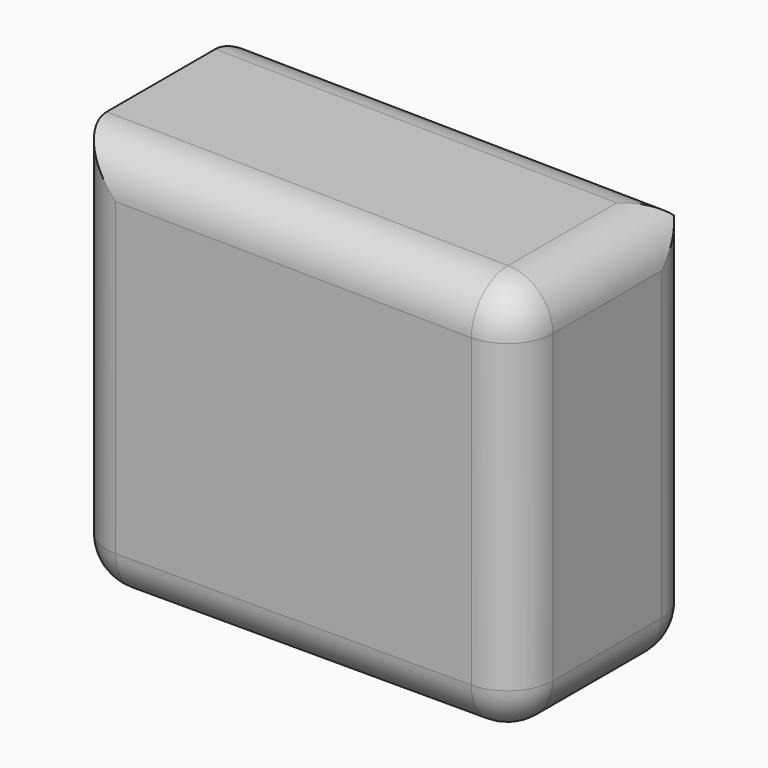
from build123d import *

# Parameters (mm, degrees)
F1_DEPTH    = 25.4
F2_R        = 5.08
F3_T1_DEPTH = 27.7897108637
F3_T6_DEPTH = 5.1816


# Not quite as in the source:
# - a fillet or chamfer that OpenCascade refuses, or shapes differently, is made with other operations: its cross-section is extruded or revolved along the edge and cut away or added


with BuildPart() as f1:
    # F0 (on Front) → F1 (new body)
    with BuildSketch(Plane.XZ):
        Polygon((-8.6416769773, 61.5346953273), (-58.7037988007, 62.1306672692), (-58.7037988007, 17.1343572438), (-8.6416769773, 17.1343572438), align=None)
    extrude(amount=F1_DEPTH)

    # F2
    f2_edges = [f1.edges().sort_by_distance(p)[0] for p in [
        (-33.672738, -25.4, 61.832681),
        (-58.703799, -25.4, 39.632512),
        (-33.672738, -25.4, 17.134357),
        (-8.641677, -25.4, 39.334526),
        (-33.672738, 0, 61.832681),
        (-58.703799, 0, 39.632512),
        (-33.672738, 0, 17.134357),
        (-8.641677, 0, 39.334526),
        (-58.703799, -12.7, 17.134357),
        (-8.641677, -12.7, 17.134357),
    ]]
    fillet(f2_edges, radius=F2_R)

    # F3: fillet of radius 5.08 on 5 edges, made by hand

    # F3_s2 → F3_t1 (cut)
    with BuildSketch(Plane.XZ.offset(-7.4697108637)):
        with BuildLine():
            ThreePointArc((-13.6612056499, 61.5944510496), (-10.1082579355, 60.0854695805), (-8.6416769773, 56.5148109818))
            Line((-8.6416769773, 56.5148109818), (-8.6416769773, 61.5346953273))
            Line((-8.6416769773, 61.5346953273), (-13.6612056499, 61.5944510496))
        make_face()
    extrude(amount=F3_T1_DEPTH, mode=Mode.SUBTRACT)


with BuildPart() as f3_tool4:
    # F3_s5 → F3_t6 (new body)
    with BuildSketch(Plane.XZ.offset(20.32)):
        Polygon((-13.7216769773, 56.5148109818), (-13.6599962234, 61.696043851), (-8.5400769773, 61.6350930142), (-8.5400769773, 56.5148109818), align=None)
    extrude(amount=F3_T6_DEPTH)

    # F3_s7 → F3_t8 (revolve, cut)
    with BuildSketch(Plane(origin=(-13.7216769773, -20.32, 56.5148109818), x_dir=(-0.711302961, 0, -0.7028855509), z_dir=(-0.7028855509, 0, 0.711302961))):
        with BuildLine():
            ThreePointArc((0, -5.08), (5.08, 0), (0, 5.08))
            Line((0, 5.08), (0, -5.08))
        make_face()
    revolve(axis=Axis((-13.7216769773, -20.32, 56.5148109818), (0, -1, 0)), mode=Mode.SUBTRACT)


with BuildPart() as f1_1:
    add(f1.part)

    # F3_t3: cut F3_tool4
    add(f3_tool4.part, mode=Mode.SUBTRACT)


solid = f1_1.part
